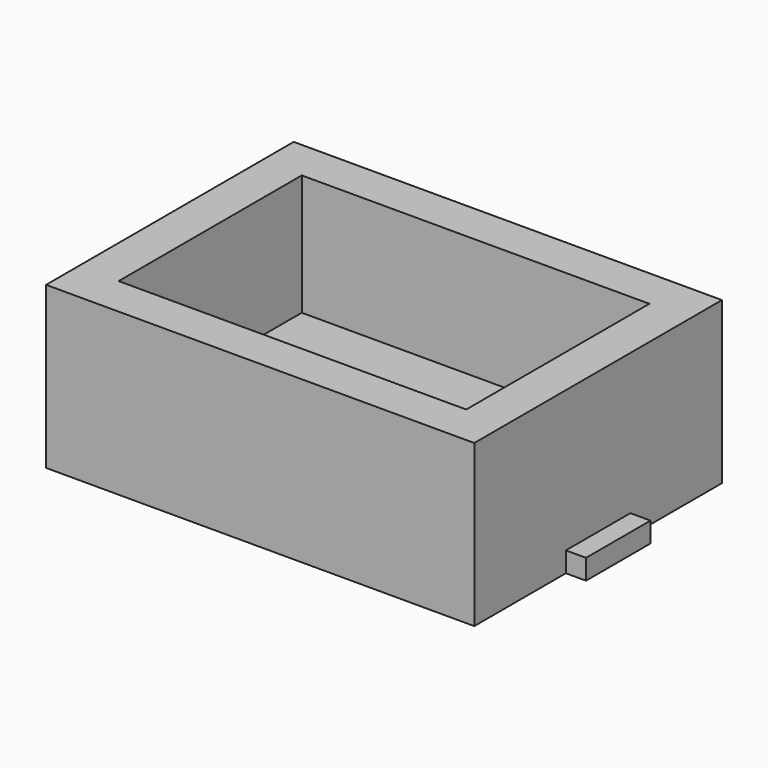
from build123d import *

# Parameters (mm, degrees)
F0_W     = 21.25
F0_H     = 15.36
F1_DEPTH = 8
F2_T     = -2
F3_W     = 4
F3_H     = 1
F4_DEPTH = 1
F5_W     = 4
F5_H     = 1
F6_DEPTH = 1


# Not quite as in the source:
# - a feature names something its author has since deleted; it is built from what else it names


with BuildPart() as f1:
    # F0 (on Top) → F1 (new body)
    with BuildSketch(Plane.XY):
        Rectangle(F0_W, F0_H)
    extrude(amount=F1_DEPTH)

    # F2
    f2_openings = [f1.faces().sort_by_distance(p)[0] for p in [
        (0, 0, 8),
    ]]
    offset(amount=F2_T, openings=f2_openings)

    # F3 (on face) → F4 (join)
    with BuildSketch(Plane(origin=(-10.625, 0, 0), x_dir=(0, -1, 0), z_dir=(-1, 0, 0))):
        with Locations((0, 0.5)):
            Rectangle(F3_W, F3_H)
    extrude(amount=F4_DEPTH)

    # F5 (on face) → F6 (join)
    with BuildSketch(Plane.YZ.offset(10.625)):
        with Locations((0, 0.5)):
            Rectangle(F5_W, F5_H)
    extrude(amount=F6_DEPTH)


solid = f1.part
